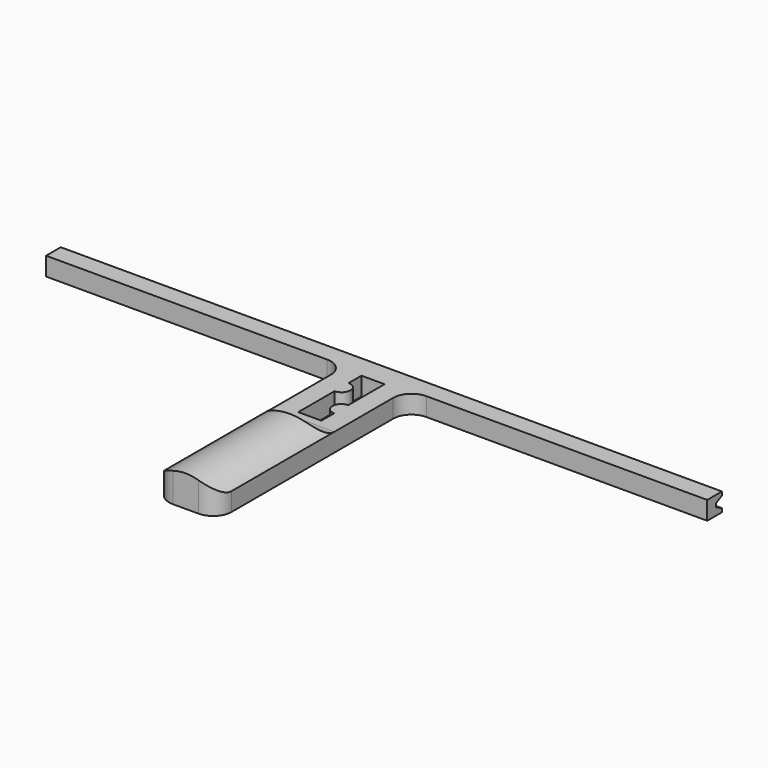
from build123d import *

# Parameters (mm, degrees)
F1_DEPTH      = 5
F3_DEPTH      = 5.001
F5_DEPTH      = 35
F6_W          = 5
F6_H          = 5
F7_DEPTH      = 90
F7_DEPTH_BACK = 90
F9_DEPTH      = 180.001
F10_T1_DEPTH  = 5
F10_T6_DEPTH  = 17.0072864353
F10_S7_R      = 12
F10_T8_DEPTH  = 11
F10_T9_DEPTH  = 30


# Not quite as in the source:
# - a fillet or chamfer that OpenCascade refuses, or shapes differently, is made with other operations: its cross-section is extruded or revolved along the edge and cut away or added


with BuildPart() as f1:
    # F0 (on Top) → F1 (new body)
    with BuildSketch(Plane.XY):
        Polygon((8.5036432176, -40), (-8.5036432176, -40), (-8.5036432176, -110), (0, -110), (8.5036432176, -110), align=None)
    extrude(amount=F1_DEPTH)

    # F2 (on face) → F3 (cut, through all)
    with BuildSketch(Plane.XY.offset(5)):
        with BuildLine():
            Line((-3.15, -67.75), (3.15, -67.75))
            Line((3.15, -67.75), (3.15, -63.4))
            ThreePointArc((3.15, -63.4), (0.75, -61), (3.15, -58.6))
            Line((3.15, -58.6), (3.15, -46.25))
            Line((3.15, -46.25), (-3.15, -46.25))
            Line((-3.15, -46.25), (-3.15, -50.6))
            ThreePointArc((-3.15, -50.6), (-0.75, -53), (-3.15, -55.4))
            Line((-3.15, -55.4), (-3.15, -67.75))
        make_face()
    extrude(amount=-F3_DEPTH, mode=Mode.SUBTRACT)

    # F4 (on face) → F5 (join)
    with BuildSketch(Plane.XZ.offset(110)):
        with BuildLine():
            ThreePointArc((8.5036432176, 5), (0, 8.5331202898), (-8.5036432176, 5))
            Line((-8.5036432176, 5), (8.5036432176, 5))
        make_face()
    extrude(amount=-F5_DEPTH)

    # F6 (on Right) → F7 (join, two sides)
    with BuildSketch(Plane.YZ) as f7_sk:
        with Locations((-42.5, 2.5)):
            Rectangle(F6_W, F6_H)
    extrude(amount=F7_DEPTH)
    extrude(f7_sk.sketch, amount=-F7_DEPTH_BACK)

    # F8 (on face) → F9 (cut, through all)
    with BuildSketch(Plane(origin=(-90, 0, 0), x_dir=(0, -1, 0), z_dir=(-1, 0, 0))):
        Polygon((40, 1), (42, 2), (42, 3), (40, 4), align=None)
    extrude(amount=-F9_DEPTH, mode=Mode.SUBTRACT)

    # F10: fillet of radius 5 on 5 edges, made by hand

    # F10_s2 → F10_t1 (join)
    with BuildSketch(Plane.XY):
        with BuildLine():
            ThreePointArc((-13.5036432176, -45), (-9.9681093117, -46.4644660941), (-8.5036432176, -50))
            Line((-8.5036432176, -50), (-8.5036432176, -45))
            Line((-8.5036432176, -45), (-13.5036432176, -45))
        make_face()
        with BuildLine():
            ThreePointArc((8.5036432176, -50), (9.9681093117, -46.4644660941), (13.5036432176, -45))
            Line((13.5036432176, -45), (8.5036432176, -45))
            Line((8.5036432176, -45), (8.5036432176, -50))
        make_face()
    extrude(amount=F10_T1_DEPTH)


with BuildPart() as f10_tool4:
    # F10_s5 → F10_t6 (new body)
    with BuildSketch(Plane.YZ.offset(-8.5036432176)):
        with BuildLine():
            ThreePointArc((-70, 5), (-73.5355339059, 6.4644660941), (-75, 10))
            Line((-75, 10), (-75, 5))
            Line((-75, 5), (-70, 5))
        make_face()
    extrude(amount=F10_T6_DEPTH)

    # F10_s7 → F10_t8 (intersect, symmetric)
    with BuildSketch(Plane.XZ.offset(72.5)):
        with Locations((0, -3.4668797102)):
            Circle(F10_S7_R)
    extrude(amount=F10_T8_DEPTH, both=True, mode=Mode.INTERSECT)


with BuildPart() as f1_1:
    add(f1.part)

    # F10_t3: union F10_tool4
    add(f10_tool4.part)

    # F10_s10 → F10_t9 (cut)
    with BuildSketch(Plane.XY.offset(-12.5)):
        with BuildLine():
            ThreePointArc((-8.5036432176, -105), (-7.0391771236, -108.5355339059), (-3.5036432176, -110))
            Line((-3.5036432176, -110), (-8.5036432176, -110))
            Line((-8.5036432176, -110), (-8.5036432176, -105))
        make_face()
        with BuildLine():
            ThreePointArc((8.5036432176, -105), (7.0391771236, -108.5355339059), (3.5036432176, -110))
            Line((3.5036432176, -110), (8.5036432176, -110))
            Line((8.5036432176, -110), (8.5036432176, -105))
        make_face()
    extrude(amount=F10_T9_DEPTH, mode=Mode.SUBTRACT)


solid = f1_1.part
